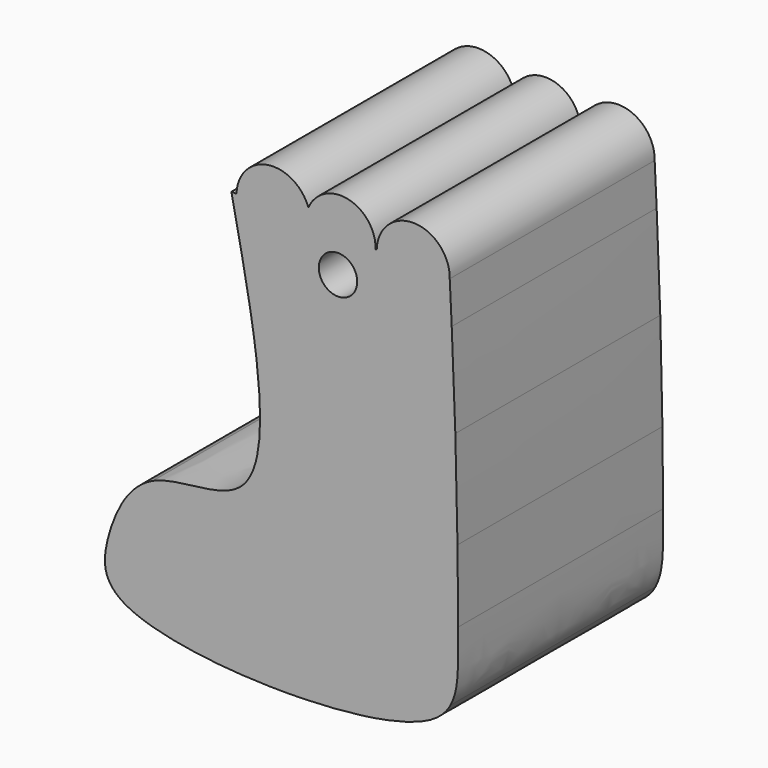
from build123d import *

# Parameters (mm, degrees)
F0_W         = 8.8834874332
F0_H         = 7.0633614465
F1_DEPTH     = 25.4
F3_D         = 3.81
F4_TEXT_SIZE = 10.8793701252
F5_DEPTH     = 12.7


# Not quite as in the source:
# - Text() gives the source's letters only with a copy of the font that has no kerning and outlines rounded to 1/6400 em; it was checked with that copy


with BuildPart() as f1:
    # F0 (on Front) → F1 (new body)
    with BuildSketch(Plane.XZ):
        with BuildLine():
            Line((17.4911456118, 45.1942725744), (16.9817954302, 45.2073328197))
            add(Edge.make_bspline(
                [(16.9817954302, 45.2073328197), (17.3464826654, 43.4358490372), (17.7111699007, 41.6643652547), (18.0519473906, 39.9250312339)],
                knots=[0, 0, 0, 0, 0.027586504, 0.027586504, 0.027586504, 0.027586504], degree=3))
            Line((18.0519473906, 39.9250312339), (23.0847798847, 40.0780397075))
            Line((23.0847798847, 40.0780397075), (32.514764863, 40.3647306731))
            Line((32.514764863, 40.3647306731), (38.8323951836, 40.5567996468))
            add(Edge.make_bspline(
                [(38.8323951836, 40.5567996468), (38.7678147825, 41.9468781146), (38.7015548335, 43.2994968341), (38.6352948844, 44.6521155536)],
                knots=[0.9590756675, 0.9590756675, 0.9590756675, 0.9590756675, 1, 1, 1, 1], degree=3))
            Line((38.6352948844, 44.6521155536), (31.3937513584, 44.8377959332))
            Line((31.3937513584, 44.8377959332), (31.2858317281, 44.8405630999))
            Line((31.2858317281, 44.8405630999), (24.8236937195, 45.0062587467))
            ThreePointArc((24.8236937195, 45.0062587467), (24.7464126591, 44.3455922006), (24.551071234, 43.7097507306))
            ThreePointArc((24.551071234, 43.7097507306), (24.3781358463, 44.3537349909), (24.3312585865, 45.0188852734))
            Line((24.3312585865, 45.0188852734), (17.4911456118, 45.1942725744))
        make_face()
        with BuildLine():
            Line((23.0847798847, 40.0780397075), (18.0519473906, 39.9250312339))
            add(Edge.make_bspline(
                [(18.0519473906, 39.9250312339), (18.6434304526, 36.9060917708), (19.1628827915, 33.9840069818), (19.4852816166, 31.3268862665)],
                knots=[0.027586504, 0.027586504, 0.027586504, 0.027586504, 0.0754680405, 0.0754680405, 0.0754680405, 0.0754680405], degree=3))
            Line((19.4852816166, 31.3268862665), (23.3508329734, 31.3268862665))
            Line((23.3508329734, 31.3268862665), (23.0847798847, 40.0780397075))
        make_face()
        with BuildLine():
            ThreePointArc((24.6178733019, 46.3150345149), (20.5876676644, 48.7232182403), (17.4911456118, 45.1942725744))
            Line((17.4911456118, 45.1942725744), (24.3312585865, 45.0188852734))
            ThreePointArc((24.3312585865, 45.0188852734), (24.4121620653, 45.6807591307), (24.6178733019, 46.3150345149))
        make_face()
        with BuildLine():
            Line((23.3508329734, 31.3268862665), (19.4852816166, 31.3268862665))
            add(Edge.make_bspline(
                [(19.4852816166, 31.3268862665), (19.9723990897, 27.3122006416), (20.0096696973, 23.9023926246), (19.1658624516, 21.6773083549)],
                knots=[0.0754680405, 0.0754680405, 0.0754680405, 0.0754680405, 0.1478130098, 0.1478130098, 0.1478130098, 0.1478130098], degree=3))
            Line((19.1658624516, 21.6773083549), (23.6442000164, 21.6773083549))
            Line((23.6442000164, 21.6773083549), (23.3508329734, 31.3268862665))
        make_face()
        Polygon((32.514764863, 40.3647306731), (23.0847798847, 40.0780397075), (23.3508329734, 31.3268862665), (32.514764863, 31.3268862665), align=None)
        with BuildLine():
            ThreePointArc((24.6178733019, 46.3150345149), (24.4121620653, 45.6807591307), (24.3312585865, 45.0188852734))
            Line((24.3312585865, 45.0188852734), (24.8236937195, 45.0062587467))
            ThreePointArc((24.8236937195, 45.0062587467), (24.7803722454, 45.6700176618), (24.6178733019, 46.3150345149))
        make_face()
        with BuildLine():
            Line((24.8236937195, 45.0062587467), (24.3312585865, 45.0188852734))
            ThreePointArc((24.3312585865, 45.0188852734), (24.3781358463, 44.3537349909), (24.551071234, 43.7097507306))
            ThreePointArc((24.551071234, 43.7097507306), (24.7464126591, 44.3455922006), (24.8236937195, 45.0062587467))
        make_face()
        with BuildLine():
            ThreePointArc((31.2858317281, 44.8405630999), (28.5595801014, 48.3261072786), (24.6178733019, 46.3150345149))
            ThreePointArc((24.6178733019, 46.3150345149), (24.7803722454, 45.6700176618), (24.8236937195, 45.0062587467))
            Line((24.8236937195, 45.0062587467), (31.2858317281, 44.8405630999))
        make_face()
        with BuildLine():
            Line((23.6442000164, 21.6773083549), (19.1658624516, 21.6773083549))
            add(Edge.make_bspline(
                [(19.1658624516, 21.6773083549), (18.8999700041, 20.9761611376), (18.5465913094, 20.3926505561), (18.0922336876, 19.9449192733)],
                knots=[0.1478130098, 0.1478130098, 0.1478130098, 0.1478130098, 0.1706096628, 0.1706096628, 0.1706096628, 0.1706096628], degree=3))
            Line((18.0922336876, 19.9449192733), (18.0922336876, 14.5258473803))
            Line((18.0922336876, 14.5258473803), (23.8616191594, 14.5258473803))
            Line((23.8616191594, 14.5258473803), (23.6442000164, 21.6773083549))
        make_face()
        Polygon((32.514764863, 31.3268862665), (23.3508329734, 31.3268862665), (23.6442000164, 21.6773083549), (32.514764863, 21.6773083549), align=None)
        with BuildLine():
            Line((38.8323951836, 40.5567996468), (32.514764863, 40.3647306731))
            Line((32.514764863, 40.3647306731), (32.514764863, 31.3268862665))
            Line((32.514764863, 31.3268862665), (39.1905121505, 31.3268862665))
            add(Edge.make_bspline(
                [(39.1905121505, 31.3268862665), (39.0873786126, 34.7657053136), (38.963339397, 37.7382551895), (38.8323951836, 40.5567996468)],
                knots=[0.8760968623, 0.8760968623, 0.8760968623, 0.8760968623, 0.9590756675, 0.9590756675, 0.9590756675, 0.9590756675], degree=3))
        make_face()
        with BuildLine():
            Line((18.0922336876, 14.5258473803), (18.0922336876, 19.9449192733))
            add(Edge.make_bspline(
                [(18.0922336876, 19.9449192733), (16.0380433262, 17.9206871668), (11.9198206578, 18.6718148997), (9.2087462544, 17.4464378506)],
                knots=[0.1706096628, 0.1706096628, 0.1706096628, 0.1706096628, 0.2736753153, 0.2736753153, 0.2736753153, 0.2736753153], degree=3))
            Line((9.2087462544, 17.4464378506), (9.2087462544, 14.5258473803))
            Line((9.2087462544, 14.5258473803), (18.0922336876, 14.5258473803))
        make_face()
        Polygon((32.514764863, 21.6773083549), (23.6442000164, 21.6773083549), (23.8616191594, 14.5258473803), (32.514764863, 14.5258473803), align=None)
        with BuildLine():
            Line((39.1905121505, 31.3268862665), (32.514764863, 31.3268862665))
            Line((32.514764863, 31.3268862665), (32.514764863, 21.6773083549))
            Line((32.514764863, 21.6773083549), (39.4045704056, 21.6773083549))
            add(Edge.make_bspline(
                [(39.4045704056, 21.6773083549), (39.355195461, 24.9426445986), (39.280878936, 28.3137536902), (39.1905121505, 31.3268862665)],
                knots=[0.8033898842, 0.8033898842, 0.8033898842, 0.8033898842, 0.8760968623, 0.8760968623, 0.8760968623, 0.8760968623], degree=3))
        make_face()
        with BuildLine():
            ThreePointArc((38.6352948844, 44.6521155536), (35.1073633112, 48.3657275064), (31.3937513584, 44.8377959332))
            Line((31.3937513584, 44.8377959332), (38.6352948844, 44.6521155536))
        make_face()
        with BuildLine():
            Line((9.2087462544, 14.5258473803), (9.2087462544, 17.4464378506))
            add(Edge.make_bspline(
                [(9.2087462544, 17.4464378506), (7.881095101, 16.8463535259), (6.8909059976, 15.772264171), (6.1572941287, 14.5258473803)],
                knots=[0.2736753153, 0.2736753153, 0.2736753153, 0.2736753153, 0.3241480107, 0.3241480107, 0.3241480107, 0.3241480107], degree=3))
            Line((6.1572941287, 14.5258473803), (9.2087462544, 14.5258473803))
        make_face()
        Polygon((23.8616191594, 14.5258473803), (18.0922336876, 14.5258473803), (18.0922336876, 7.4624859338), (24.0763598953, 7.4624859338), align=None)
        with Locations((13.650489971, 10.9941666571)):
            Rectangle(F0_W, F0_H)
        Polygon((32.514764863, 14.5258473803), (23.8616191594, 14.5258473803), (24.0763598953, 7.4624859338), (32.514764863, 7.4624859338), align=None)
        with BuildLine():
            Line((39.4045704056, 21.6773083549), (32.514764863, 21.6773083549))
            Line((32.514764863, 21.6773083549), (32.514764863, 14.5258473803))
            Line((32.514764863, 14.5258473803), (39.4702205591, 14.5258473803))
            add(Edge.make_bspline(
                [(39.4702205591, 14.5258473803), (39.4658796197, 16.7051044992), (39.4426379535, 19.1597694509), (39.4045704056, 21.6773083549)],
                knots=[0.747333591, 0.747333591, 0.747333591, 0.747333591, 0.8033898842, 0.8033898842, 0.8033898842, 0.8033898842], degree=3))
        make_face()
        with BuildLine():
            Line((9.2087462544, 14.5258473803), (6.1572941287, 14.5258473803))
            add(Edge.make_bspline(
                [(6.1572941287, 14.5258473803), (5.5155959091, 13.4355931608), (4.5618813514, 10.8186738094), (4.2600951947, 8.5229474358), (4.7670030035, 7.4624859338)],
                knots=[0.3241480107, 0.3241480107, 0.3241480107, 0.3241480107, 0.3682970221, 0.4186852087, 0.4186852087, 0.4186852087, 0.4186852087], degree=3))
            Line((4.7670030035, 7.4624859338), (9.2087462544, 7.4624859338))
            Line((9.2087462544, 7.4624859338), (9.2087462544, 14.5258473803))
        make_face()
        with BuildLine():
            Line((24.0763598953, 7.4624859338), (18.0922336876, 7.4624859338))
            Line((18.0922336876, 7.4624859338), (18.0922336876, 3.3729356904))
            add(Edge.make_bspline(
                [(18.0922336876, 3.3729356904), (20.099146483, 3.2533127163), (22.1774787817, 3.2204141732), (24.2036201482, 3.2765770024)],
                knots=[0.5258084959, 0.5258084959, 0.5258084959, 0.5258084959, 0.5574700226, 0.5574700226, 0.5574700226, 0.5574700226], degree=3))
            Line((24.2036201482, 3.2765770024), (24.0763598953, 7.4624859338))
        make_face()
        with BuildLine():
            Line((18.0922336876, 3.3729356904), (18.0922336876, 7.4624859338))
            Line((18.0922336876, 7.4624859338), (9.2087462544, 7.4624859338))
            Line((9.2087462544, 7.4624859338), (9.2087462544, 4.6875571956))
            add(Edge.make_bspline(
                [(9.2087462544, 4.6875571956), (11.5864606855, 4.0146036507), (14.7396972954, 3.5727651873), (18.0922336876, 3.3729356904)],
                knots=[0.4729180959, 0.4729180959, 0.4729180959, 0.4729180959, 0.5258084959, 0.5258084959, 0.5258084959, 0.5258084959], degree=3))
        make_face()
        with BuildLine():
            Line((32.514764863, 7.4624859338), (24.0763598953, 7.4624859338))
            Line((24.0763598953, 7.4624859338), (24.2036201482, 3.2765770024))
            add(Edge.make_bspline(
                [(24.2036201482, 3.2765770024), (27.2271407945, 3.3603862944), (30.1344412871, 3.6425198147), (32.514764863, 4.1307432053)],
                knots=[0.5574700226, 0.5574700226, 0.5574700226, 0.5574700226, 0.6047171108, 0.6047171108, 0.6047171108, 0.6047171108], degree=3))
            Line((32.514764863, 4.1307432053), (32.514764863, 7.4624859338))
        make_face()
        with BuildLine():
            Line((39.4702205591, 14.5258473803), (32.514764863, 14.5258473803))
            Line((32.514764863, 14.5258473803), (32.514764863, 7.4624859338))
            Line((32.514764863, 7.4624859338), (38.7136678135, 7.4624859338))
            add(Edge.make_bspline(
                [(38.7136678135, 7.4624859338), (39.4293060448, 8.7850444348), (39.4690280381, 10.9759851586), (39.4716651821, 13.8006115358), (39.4702205591, 14.5258473803)],
                knots=[0.6714867917, 0.6714867917, 0.6714867917, 0.6714867917, 0.7286785949, 0.747333591, 0.747333591, 0.747333591, 0.747333591], degree=3))
        make_face()
        with BuildLine():
            Line((9.2087462544, 7.4624859338), (4.7670030035, 7.4624859338))
            add(Edge.make_bspline(
                [(4.7670030035, 7.4624859338), (5.0628283766, 6.843613204), (6.0278449875, 5.8047185865), (8.0926387159, 5.0034439626), (9.2087462544, 4.6875571956)],
                knots=[0.4186852087, 0.4186852087, 0.4186852087, 0.4186852087, 0.4480911556, 0.4729180959, 0.4729180959, 0.4729180959, 0.4729180959], degree=3))
            Line((9.2087462544, 4.6875571956), (9.2087462544, 7.4624859338))
        make_face()
        with BuildLine():
            Line((38.7136678135, 7.4624859338), (32.514764863, 7.4624859338))
            Line((32.514764863, 7.4624859338), (32.514764863, 4.1307432053))
            add(Edge.make_bspline(
                [(32.514764863, 4.1307432053), (33.9406417249, 4.4232019463), (36.8584099283, 5.2876246741), (38.2323268238, 6.572928068), (38.7136678135, 7.4624859338)],
                knots=[0.6047171108, 0.6047171108, 0.6047171108, 0.6047171108, 0.6330193679, 0.6714867917, 0.6714867917, 0.6714867917, 0.6714867917], degree=3))
        make_face()
    extrude(amount=F1_DEPTH)

    # F3 (through all)
    with Locations(Plane(origin=(0, 0, 0), x_dir=(1, 0, 0), z_dir=(0, 1, 0))):
        with Locations((27.5558941066, -41.4037778974)):
            Hole(F3_D / 2)

    # F4 (on Front) → F5 (join)
    with BuildSketch(Plane.XZ):
        with Locations((5.734984763, 6.7141260952)):
            Text('Kaitlyn', F4_TEXT_SIZE, font='Open Sans', font_style=FontStyle.ITALIC, text_align=(TextAlign.LEFT, TextAlign.BOTTOM))
    extrude(amount=F5_DEPTH)


solid = f1.part
